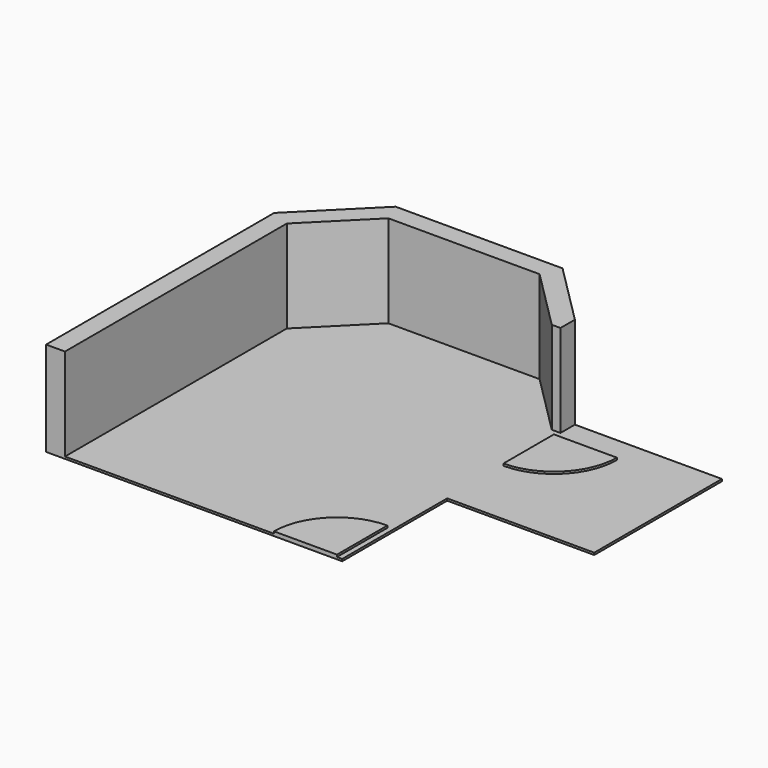
from build123d import *

# Parameters (mm, degrees)
F1_DEPTH = 25.4
F2_DEPTH = 25.4
F3_DEPTH = 1117.6


# Not quite as in the source:
# - the program builds the solid bodies; features that only make, move or delete a surface that nothing else refers to are left out


with BuildPart() as f1:
    # F0 (on Top) → F1 (new body)
    with BuildSketch(Plane.XY):
        with BuildLine():
            Line((-63.5, 0), (0, 0))
            Line((0, 0), (0, 1586.688150761))
            Line((0, 1586.688150761), (0, 2437.588150761))
            Line((0, 2437.588150761), (0, 3199.588150761))
            Line((0, 3199.588150761), (0, 3298.9184632736))
            Line((0, 3298.9184632736), (-105.1195328711, 3298.9184632736))
            Line((-105.1195328711, 3298.9184632736), (-841.5005347987, 4035.2994652013))
            Line((-841.5005347987, 4035.2994652013), (-2670.3005347987, 4035.2994652013))
            Line((-2670.3005347987, 4035.2994652013), (-3352.8, 3352.8))
            Line((-3352.8, 3352.8), (-3352.8, 0))
            Line((-3352.8, 0), (-825.5, 0))
            ThreePointArc((-825.5, 0), (-602.3153672642, 538.8153672642), (-63.5, 762))
            Line((-63.5, 762), (-63.5, 0))
        make_face()
        with BuildLine():
            Line((-825.5, 0), (-63.5, 0))
            Line((-63.5, 0), (-63.5, 762))
            ThreePointArc((-63.5, 762), (-602.3153672642, 538.8153672642), (-825.5, 0))
        make_face()
        with BuildLine():
            Line((0, 2437.588150761), (0, 1586.688150761))
            Line((0, 1586.688150761), (1778, 1586.688150761))
            Line((1778, 1586.688150761), (1778, 3517.088150761))
            Line((1778, 3517.088150761), (0, 3517.088150761))
            Line((0, 3517.088150761), (0, 3298.9184632736))
            Line((0, 3298.9184632736), (0, 3199.588150761))
            Line((0, 3199.588150761), (762, 3199.588150761))
            ThreePointArc((762, 3199.588150761), (538.8153672641, 2660.7727834969), (0, 2437.588150761))
        make_face()
        Polygon((-3581.4, 0), (-3352.8, 0), (-3352.8, 3352.8), (-2670.3005347987, 4035.2994652013), (-841.5005347987, 4035.2994652013), (-105.1195328711, 3298.9184632736), (0, 3298.9184632736), (0, 3517.088150761), (-746.8113144403, 4263.8994652013), (-2764.9897551572, 4263.8994652013), (-3581.4, 3447.4892203585), align=None)
        with BuildLine():
            Line((0, 3199.588150761), (0, 2437.588150761))
            ThreePointArc((0, 2437.588150761), (538.8153672641, 2660.7727834969), (762, 3199.588150761))
            Line((762, 3199.588150761), (0, 3199.588150761))
        make_face()
    extrude(amount=-F1_DEPTH)

    # F0 (on Top) → F2 (join)
    with BuildSketch(Plane.XY):
        with BuildLine():
            Line((0, 3199.588150761), (0, 2437.588150761))
            ThreePointArc((0, 2437.588150761), (538.8153672641, 2660.7727834969), (762, 3199.588150761))
            Line((762, 3199.588150761), (0, 3199.588150761))
        make_face()
        with BuildLine():
            Line((-825.5, 0), (-63.5, 0))
            Line((-63.5, 0), (-63.5, 762))
            ThreePointArc((-63.5, 762), (-602.3153672642, 538.8153672642), (-825.5, 0))
        make_face()
    extrude(amount=F2_DEPTH)

    # F0 (on Top) → F3 (join)
    with BuildSketch(Plane.XY):
        Polygon((-3581.4, 0), (-3352.8, 0), (-3352.8, 3352.8), (-2670.3005347987, 4035.2994652013), (-841.5005347987, 4035.2994652013), (-105.1195328711, 3298.9184632736), (0, 3298.9184632736), (0, 3517.088150761), (-746.8113144403, 4263.8994652013), (-2764.9897551572, 4263.8994652013), (-3581.4, 3447.4892203585), align=None)
    extrude(amount=F3_DEPTH)


solid = f1.part
